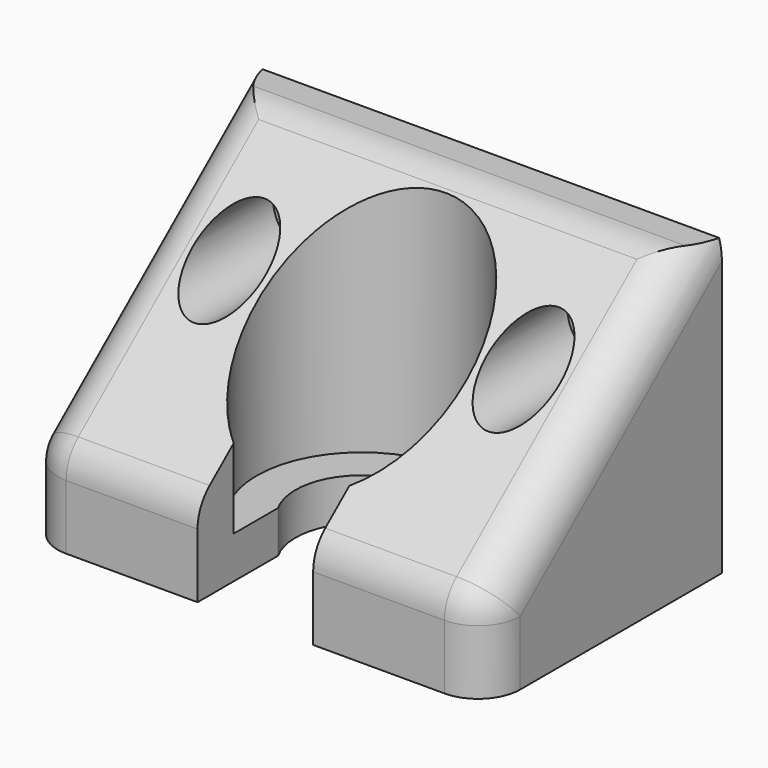
from build123d import *

# Parameters (mm, degrees)
F1_DEPTH     = 27.94
F2_R         = 12.7
F3_DEPTH     = 30.48
F4_R         = 8.0083112146
F5_DEPTH     = 50.8
F6_W         = 13.97
F6_H         = 30.48
F7_DEPTH     = 19.05
F8_T1_DEPTH  = 21.823361814
F8_T3_DEPTH  = 21.823361814
F8_T5_DEPTH  = 20.4806552744
F8_T7_DEPTH  = 49.996723628
F8_T9_DEPTH  = 65.0760683536
F8_T14_DEPTH = 5.08
F8_T20_DEPTH = 5.08
F9_R         = 2.54
F10_DEPTH    = 20.321
F12_R        = 4.445
F13_DEPTH    = 25.4


# Not quite as in the source:
# - a fillet or chamfer that OpenCascade refuses, or shapes differently, is made with other operations: its cross-section is extruded or revolved along the edge and cut away or added


with BuildPart() as f1:
    # F0 (on Right) → F1 (new body, symmetric)
    with BuildSketch(Plane.YZ):
        Polygon((-16.0675346851, 10.16), (-16.0675346851, 0), (19.4924653149, 0), (19.4924653149, 35.56), (14.4124653149, 35.56), align=None)
    extrude(amount=F1_DEPTH, both=True)

    # F2 (on face) → F3 (cut)
    with BuildSketch(Plane.XY.offset(35.56)):
        Circle(F2_R)
    extrude(amount=-F3_DEPTH, mode=Mode.SUBTRACT)

    # F4 (on face) → F5 (cut)
    with BuildSketch(Plane.XY.offset(5.08)):
        Circle(F4_R)
    extrude(amount=-F5_DEPTH, mode=Mode.SUBTRACT)

    # F6 (on face) → F7 (cut)
    with BuildSketch(Plane.XZ.offset(16.0675346851)):
        Rectangle(F6_W, F6_H)
    extrude(amount=-F7_DEPTH, mode=Mode.SUBTRACT)

    # F8: fillet of radius 5.08 on 7 edges, made by hand

    # F8_s2 → F8_t1 (cut)
    with BuildSketch(Plane.YZ.offset(-22.86)):
        with BuildLine():
            ThreePointArc((-16.0675346851, 7.7806552744), (-15.587928945, 9.9353646873), (-14.2396714354, 11.6832193748))
            Line((-14.2396714354, 11.6832193748), (-16.0675346851, 10.16))
            Line((-16.0675346851, 10.16), (-16.0675346851, 7.7806552744))
        make_face()
    extrude(amount=F8_T1_DEPTH, mode=Mode.SUBTRACT)

    # F8_s4 → F8_t3 (cut)
    with BuildSketch(Plane.YZ.offset(1.036638186)):
        with BuildLine():
            ThreePointArc((-16.0675346851, 7.7806552744), (-15.587928945, 9.9353646873), (-14.2396714354, 11.6832193748))
            Line((-14.2396714354, 11.6832193748), (-16.0675346851, 10.16))
            Line((-16.0675346851, 10.16), (-16.0675346851, 7.7806552744))
        make_face()
    extrude(amount=F8_T3_DEPTH, mode=Mode.SUBTRACT)

    # F8_s6 → F8_t5 (cut)
    with BuildSketch(Plane.XY.offset(-12.7)):
        with BuildLine():
            ThreePointArc((27.94, -10.9875346851), (26.4521024484, -14.5796371336), (22.86, -16.0675346851))
            Line((22.86, -16.0675346851), (27.94, -16.0675346851))
            Line((27.94, -16.0675346851), (27.94, -10.9875346851))
        make_face()
        with BuildLine():
            ThreePointArc((-22.86, -16.0675346851), (-26.4521024484, -14.5796371336), (-27.94, -10.9875346851))
            Line((-27.94, -10.9875346851), (-27.94, -16.0675346851))
            Line((-27.94, -16.0675346851), (-22.86, -16.0675346851))
        make_face()
    extrude(amount=F8_T5_DEPTH, mode=Mode.SUBTRACT)

    # F8_s8 → F8_t7 (cut)
    with BuildSketch(Plane(origin=(0, 35.7506520761, 29.7922100634), x_dir=(1, 0, 0), z_dir=(0, -0.7682212796, -0.6401843997))):
        with BuildLine():
            ThreePointArc((27.94, 13.0113132472), (26.4521024484, 16.6034156956), (22.86, 18.0913132472))
            Line((22.86, 18.0913132472), (27.94, 18.0913132472))
            Line((27.94, 18.0913132472), (27.94, 13.0113132472))
        make_face()
        with BuildLine():
            ThreePointArc((-27.94, 13.0113132472), (-26.4521024484, 16.6034156956), (-22.86, 18.0913132472))
            Line((-22.86, 18.0913132472), (-27.94, 18.0913132472))
            Line((-27.94, 18.0913132472), (-27.94, 13.0113132472))
        make_face()
    extrude(amount=F8_T7_DEPTH, mode=Mode.SUBTRACT)

    # F8_s10 → F8_t9 (cut)
    with BuildSketch(Plane.YZ.offset(-32.5380341768)):
        with BuildLine():
            ThreePointArc((16.2516789856, 35.56), (14.5223186457, 35.2565796146), (12.9995422353, 34.3825641004))
            Line((12.9995422353, 34.3825641004), (14.4124653149, 35.56))
            Line((14.4124653149, 35.56), (16.2516789856, 35.56))
        make_face()
    extrude(amount=F8_T9_DEPTH, mode=Mode.SUBTRACT)


with BuildPart() as f8_tool12:
    # F8_s13 → F8_t14 (new body)
    with BuildSketch(Plane.YZ.offset(-22.86)):
        Polygon((-10.9875346851, 7.7806552744), (-14.2396714354, 11.6832193748), (-16.0675346851, 10.16), (-16.0675346851, 7.7806552744), align=None)
    extrude(amount=-F8_T14_DEPTH)

    # F8_s15 → F8_t16 (revolve, cut)
    with BuildSketch(Plane(origin=(-22.86, -10.9875346851, 7.7806552744), x_dir=(0, 0.9055894212, -0.4241553962), z_dir=(0, 0.4241553962, 0.9055894212))):
        with BuildLine():
            ThreePointArc((0, -5.08), (5.08, 0), (0, 5.08))
            Line((0, 5.08), (0, -5.08))
        make_face()
    revolve(axis=Axis((-22.86, -10.9875346851, 7.7806552744), (-1, 0, 0)), mode=Mode.SUBTRACT)


with BuildPart() as f1_1:
    add(f1.part)

    # F8_t11: cut F8_tool12
    add(f8_tool12.part, mode=Mode.SUBTRACT)


with BuildPart() as f8_tool18:
    # F8_s19 → F8_t20 (new body)
    with BuildSketch(Plane.YZ.offset(22.86)):
        Polygon((-10.9875346851, 7.7806552744), (-16.0675346851, 7.7806552744), (-16.0675346851, 10.16), (-14.2396714354, 11.6832193748), align=None)
    extrude(amount=F8_T20_DEPTH)

    # F8_s21 → F8_t22 (revolve, cut)
    with BuildSketch(Plane(origin=(22.86, -10.9875346851, 7.7806552744), x_dir=(0, 0.9055894212, -0.4241553962), z_dir=(0, -0.4241553962, -0.9055894212))):
        with BuildLine():
            ThreePointArc((0, -5.08), (5.08, 0), (0, 5.08))
            Line((0, 5.08), (0, -5.08))
        make_face()
    revolve(axis=Axis((22.86, -10.9875346851, 7.7806552744), (1, 0, 0)), mode=Mode.SUBTRACT)


with BuildPart() as f1_2:
    add(f1_1.part)

    # F8_t17: cut F8_tool18
    add(f8_tool18.part, mode=Mode.SUBTRACT)

    # F9 (on face) → F10 (cut, through all)
    with BuildSketch(Plane(origin=(0, 19.4924653149, 0), x_dir=(-1, 0, 0), z_dir=(0, 1, 0))):
        with Locations((-17.78, 25.4)):
            Circle(F9_R)
        with Locations((17.78, 25.4)):
            Circle(F9_R)
    extrude(amount=-F10_DEPTH, mode=Mode.SUBTRACT)

    # F12 (on offset) → F13 (cut)
    with BuildSketch(Plane(origin=(0, 14.4124653149, 0), x_dir=(-1, 0, 0), z_dir=(0, 1, 0))):
        with Locations((-17.78, 25.4)):
            Circle(F12_R)
        with Locations((17.78, 25.4)):
            Circle(F12_R)
    extrude(amount=-F13_DEPTH, mode=Mode.SUBTRACT)


solid = f1_2.part
